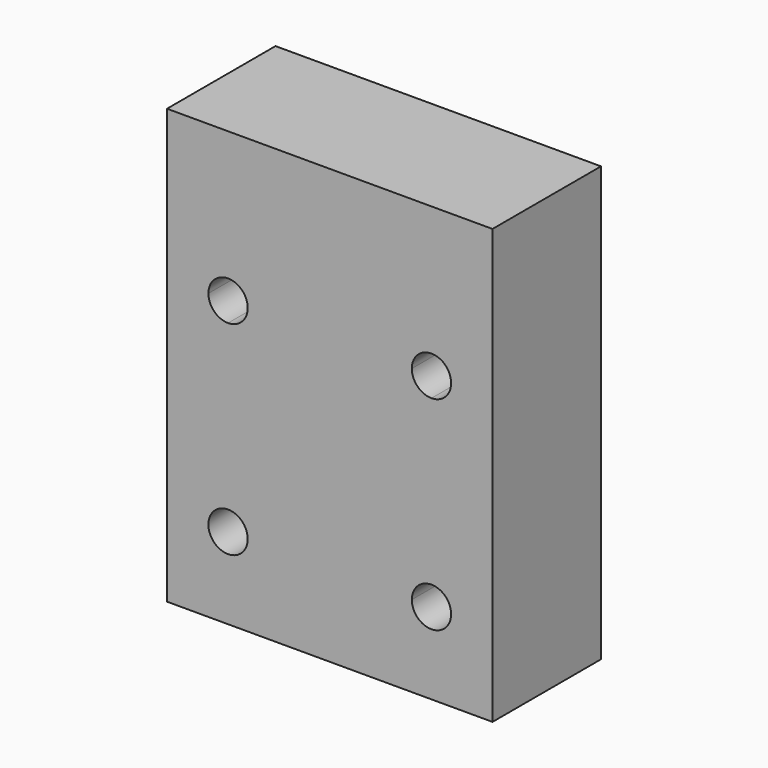
from build123d import *

# Parameters (mm, degrees)
F1_DEPTH = 10


# Not quite as in the source:
# - a feature names something its author has since deleted; it is built from what else it names


with BuildPart() as f1:
    # F0 (on Front) → F1 (new body)
    with BuildSketch(Plane.XZ):
        with BuildLine():
            Line((-0.4689496755, 31.1130427234), (-12.4689496755, 31.1130427234))
            Line((-12.4689496755, 31.1130427234), (-12.4689496755, 20.1130427234))
            Line((-12.4689496755, 20.1130427234), (-6.4189496755, 20.1130427234))
            ThreePointArc((-6.4189496755, 20.1130427234), (-4.9689496755, 21.5630427234), (-3.5189496755, 20.1130427234))
            ThreePointArc((-3.5189496755, 20.1130427234), (-3.9436448428, 19.0877378907), (-4.9689496755, 18.6630427234))
            Line((-4.9689496755, 18.6630427234), (-4.9689496755, 13.4656252339))
            Line((-4.9689496755, 13.4656252339), (-0.4689496755, 13.4656252339))
            Line((-0.4689496755, 13.4656252339), (-0.4689496755, 31.1130427234))
        make_face()
        with BuildLine():
            Line((-12.4689496755, 31.1130427234), (-24.4689496755, 31.1130427234))
            Line((-24.4689496755, 31.1130427234), (-24.4689496755, 20.1130427234))
            Line((-24.4689496755, 20.1130427234), (-21.4189496755, 20.1130427234))
            ThreePointArc((-21.4189496755, 20.1130427234), (-19.9689496755, 21.5630427234), (-18.5189496755, 20.1130427234))
            Line((-18.5189496755, 20.1130427234), (-12.4689496755, 20.1130427234))
            Line((-12.4689496755, 20.1130427234), (-12.4689496755, 31.1130427234))
        make_face()
        with BuildLine():
            Line((-6.4189496755, 20.1130427234), (-12.4689496755, 20.1130427234))
            Line((-12.4689496755, 20.1130427234), (-18.5189496755, 20.1130427234))
            ThreePointArc((-18.5189496755, 20.1130427234), (-18.9436448428, 19.0877378907), (-19.9689496755, 18.6630427234))
            Line((-19.9689496755, 18.6630427234), (-19.9689496755, 6.5630427234))
            ThreePointArc((-19.9689496755, 6.5630427234), (-18.9436448428, 6.1383475561), (-18.5189496755, 5.1130427234))
            Line((-18.5189496755, 5.1130427234), (-6.4189496755, 5.1130427234))
            ThreePointArc((-6.4189496755, 5.1130427234), (-5.9942545082, 6.1383475561), (-4.9689496755, 6.5630427234))
            Line((-4.9689496755, 6.5630427234), (-4.9689496755, 13.4656252339))
            Line((-4.9689496755, 13.4656252339), (-4.9689496755, 18.6630427234))
            ThreePointArc((-4.9689496755, 18.6630427234), (-5.9942545082, 19.0877378907), (-6.4189496755, 20.1130427234))
        make_face()
        with BuildLine():
            Line((-21.4189496755, 20.1130427234), (-24.4689496755, 20.1130427234))
            Line((-24.4689496755, 20.1130427234), (-24.4689496755, -0.8869572766))
            Line((-24.4689496755, -0.8869572766), (-0.4689496755, -0.8869572766))
            Line((-0.4689496755, -0.8869572766), (-0.4689496755, 13.4656252339))
            Line((-0.4689496755, 13.4656252339), (-4.9689496755, 13.4656252339))
            Line((-4.9689496755, 13.4656252339), (-4.9689496755, 6.5630427234))
            ThreePointArc((-4.9689496755, 6.5630427234), (-3.9436448428, 6.1383475561), (-3.5189496755, 5.1130427234))
            ThreePointArc((-3.5189496755, 5.1130427234), (-4.9689496755, 3.6630427234), (-6.4189496755, 5.1130427234))
            Line((-6.4189496755, 5.1130427234), (-18.5189496755, 5.1130427234))
            ThreePointArc((-18.5189496755, 5.1130427234), (-20.9942545082, 4.0877378907), (-19.9689496755, 6.5630427234))
            Line((-19.9689496755, 6.5630427234), (-19.9689496755, 18.6630427234))
            ThreePointArc((-19.9689496755, 18.6630427234), (-20.9942545082, 19.0877378907), (-21.4189496755, 20.1130427234))
        make_face()
    extrude(amount=F1_DEPTH)


solid = f1.part
